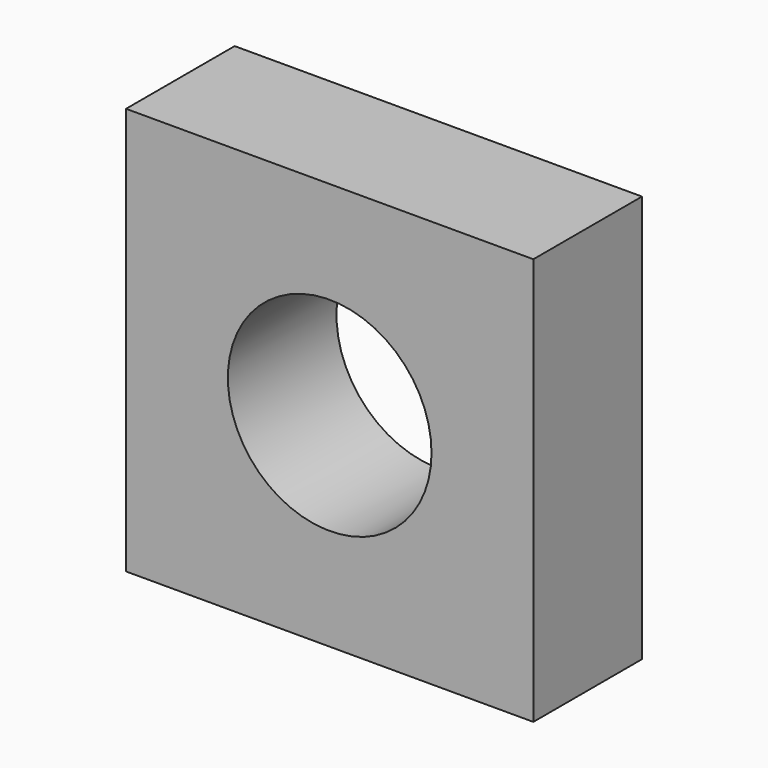
from build123d import *

# Parameters (mm, degrees)
F0_W     = 76.2
F0_H     = 76.2
F0_R     = 19.05
F1_DEPTH = 25.4


# Not quite as in the source:
# - the program builds the solid bodies; features that only make, move or delete a surface that nothing else refers to are left out


with BuildPart() as f1:
    # F0 (on Front) → F1 (new body)
    with BuildSketch(Plane.XZ):
        Rectangle(F0_W, F0_H)
        Circle(F0_R, mode=Mode.SUBTRACT)
    extrude(amount=F1_DEPTH)


solid = f1.part
